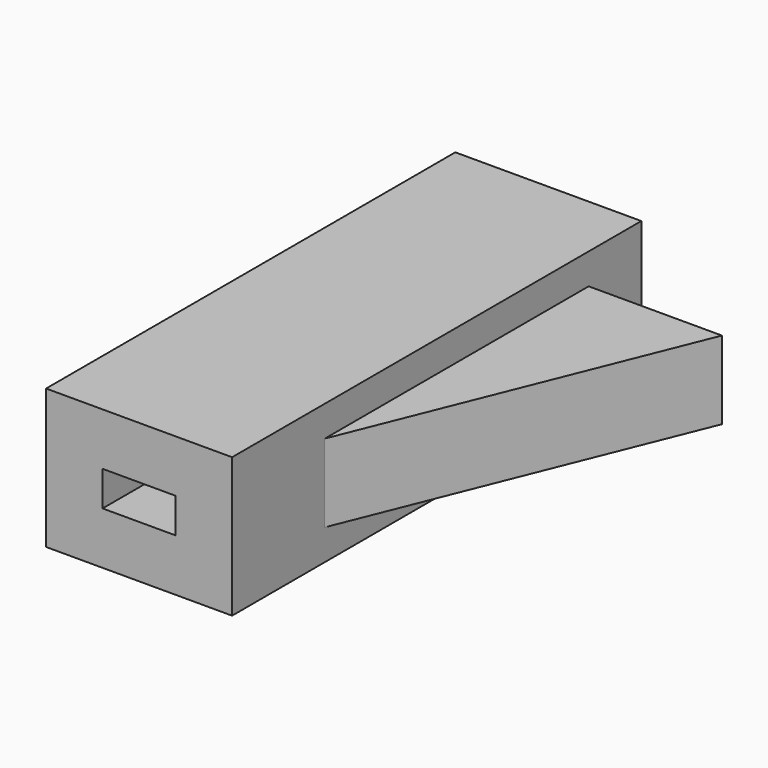
from build123d import *

# Parameters (mm, degrees)
F0_W         = 40
F0_H         = 110
F1_DEPTH     = 30
F2_W         = 81.6846340895
F2_H         = 16.7890458554
F3_DEPTH     = 30
F4_T4_DEPTH  = 457.5971749756
F5_W         = 15.7
F5_H         = 7.5
F6_DEPTH     = 12
F7_TEXT_SIZE = 4.9077603961
F8_DEPTH     = 2.5


# Not quite as in the source:
# - a fillet or chamfer that OpenCascade refuses, or shapes differently, is made with other operations: its cross-section is extruded or revolved along the edge and cut away or added
# - Text() gives the source's letters only with a copy of the font that has no kerning and outlines rounded to 1/6400 em; it was checked with that copy


with BuildPart() as f1:
    # F0 (on Top) → F1 (new body)
    with BuildSketch(Plane.XY):
        Rectangle(F0_W, F0_H)
    extrude(amount=F1_DEPTH)

    # F2 (on face) → F3 (join)
    with BuildSketch(Plane.YZ.offset(20)):
        with Locations((0, 15)):
            Rectangle(F2_W, F2_H)
    extrude(amount=F3_DEPTH)

    # F4: chamfer of 85 x 34.342229196 on 1 edges, made by hand


with BuildPart() as f4_tool2:
    # F4_s3 → F4_t4 (new body)
    with BuildSketch(Plane.XY.offset(243.7985874878)):
        Polygon((15.657770804, -40.8423170447), (50, 44.1576829553), (50, -40.8423170447), align=None)
    extrude(amount=-F4_T4_DEPTH)

    split(bisect_by=Plane.YZ.offset(20), keep=Keep.TOP)


with BuildPart() as f1_1:
    add(f1.part)

    # F4_t1: cut F4_tool2
    add(f4_tool2.part, mode=Mode.SUBTRACT)

    # F5 (on face) → F6 (cut)
    with BuildSketch(Plane.XZ.offset(55)):
        with Locations((0, 15)):
            Rectangle(F5_W, F5_H)
    extrude(amount=-F6_DEPTH, mode=Mode.SUBTRACT)

    # F7 (on face) → F8 (cut)
    with BuildSketch(Plane(origin=(0, 0, 0), x_dir=(1, 0, 0), z_dir=(0, 0, -1))):
        with Locations((0, -52.5)):
            Text('ReNew', F7_TEXT_SIZE, font='Open Sans', font_style=FontStyle.BOLD, text_align=(TextAlign.LEFT, TextAlign.BOTTOM))
    extrude(amount=-F8_DEPTH, mode=Mode.SUBTRACT)


solid = f1_1.part
